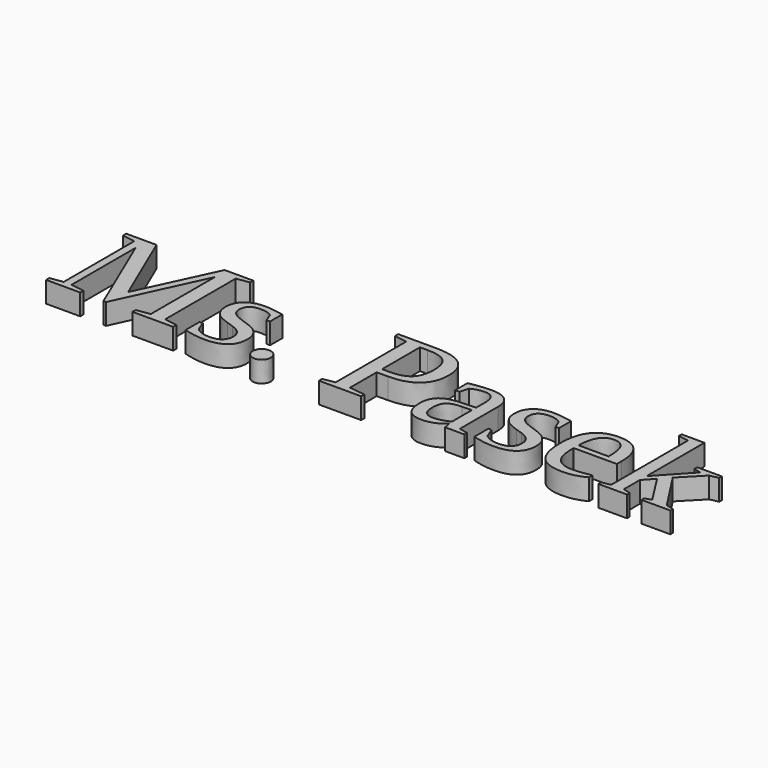
from build123d import *

# Parameters (mm, degrees)
F0_TEXT_SIZE = 23.1237553343
F1_DEPTH     = 3.175


# Not quite as in the source:
# - Text() gives the source's letters only with a copy of the font that has no kerning and outlines rounded to 1/6400 em; it was checked with that copy


with BuildPart() as f1:
    # F0 (on Top) → F1 (new body)
    with BuildSketch(Plane.XY):
        with Locations((0, 0)):
            Text('Ms. Pasek', F0_TEXT_SIZE, font='Tinos', text_align=(TextAlign.LEFT, TextAlign.BOTTOM))
    extrude(amount=F1_DEPTH)


solid = f1.part
